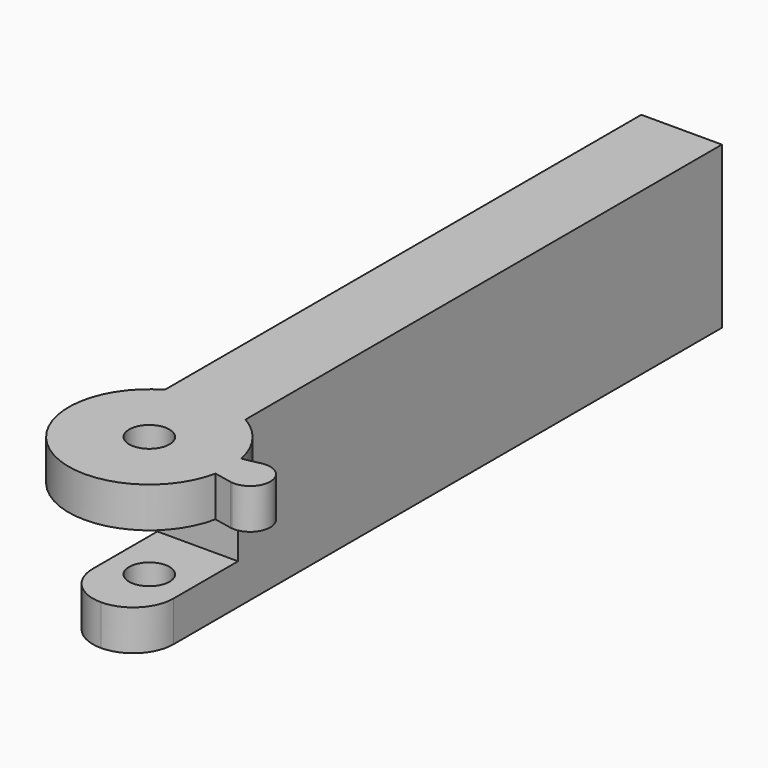
from build123d import *

# Parameters (mm, degrees)
F0_W      = 12.7
F0_H      = 114.3
F1_DEPTH  = 25.4
F2_W      = 19.05
F2_H      = 12.7
F3_DEPTH  = 12.701
F4_R      = 6.34999
F5_R      = 3.175
F6_DEPTH  = 25.401
F8_DEPTH  = 6.35
F10_DEPTH = 6.35


# Not quite as in the source:
# - a fillet or chamfer is up to 0.001 mm smaller than in the source, because OpenCascade refuses the exact size


with BuildPart() as f1:
    # F0 (on Top) → F1 (new body)
    with BuildSketch(Plane.XY):
        with Locations((6.35, 57.15)):
            Rectangle(F0_W, F0_H)
    extrude(amount=F1_DEPTH)

    # F2 (on face) → F3 (cut, through all)
    with BuildSketch(Plane.YZ.offset(12.7)):
        with Locations((9.525, 12.7)):
            Rectangle(F2_W, F2_H)
    extrude(amount=-F3_DEPTH, mode=Mode.SUBTRACT)

    # F4 (radius 6.35 in the source; OpenCascade refuses exactly that, so slightly less here)
    f4_edges = [f1.edges().sort_by_distance(p)[0] for p in [
        (12.7, 0, 22.225),
        (12.7, 0, 3.175),
        (0, 0, 3.175),
        (0, 0, 22.225),
    ]]
    fillet(f4_edges, radius=F4_R)

    # F5 (on face) → F6 (cut, through all)
    with BuildSketch(Plane.XY.offset(25.4)):
        with Locations((6.35, 9.525)):
            Circle(F5_R)
    extrude(amount=-F6_DEPTH, mode=Mode.SUBTRACT)

    # F7 (on face) → F8 (join, through all)
    with BuildSketch(Plane.XY.offset(25.4)):
        with BuildLine():
            Line((0, 6.35), (0, 20.5235226281))
            ThreePointArc((0, 20.5235226281), (6.35, -3.175), (12.7, 20.5235226281))
            Line((12.7, 20.5235226281), (12.7, 6.35))
            ThreePointArc((12.7, 6.35), (6.35, 0), (0, 6.35))
        make_face()
    extrude(amount=-F8_DEPTH)

    # F9 (on face) → F10 (join, through all)
    with BuildSketch(Plane.XY.offset(25.4)):
        with BuildLine():
            ThreePointArc((21.59, 12.6358519733), (21.7481397779, 12.663985398), (21.9075, 12.6840851128))
            ThreePointArc((21.9075, 12.6840851128), (21.9058819686, 12.6920429708), (21.9042598667, 12.7))
            Line((21.9042598667, 12.7), (21.59, 12.6358519733))
        make_face()
        with BuildLine():
            ThreePointArc((21.9075, 6.3659148872), (25.4, 9.525), (21.9075, 12.6840851128))
            ThreePointArc((21.9075, 12.6840851128), (21.7481397779, 12.663985398), (21.59, 12.6358519733))
            Line((21.59, 12.6358519733), (18.7934078933, 12.065))
            ThreePointArc((18.7934078933, 12.065), (19.05, 9.525), (18.7934078933, 6.985))
            Line((18.7934078933, 6.985), (21.59, 6.4141480267))
            ThreePointArc((21.59, 6.4141480267), (21.7481397779, 6.386014602), (21.9075, 6.3659148872))
        make_face()
        with BuildLine():
            ThreePointArc((21.9042598667, 6.35), (21.9058819686, 6.3579570292), (21.9075, 6.3659148872))
            ThreePointArc((21.9075, 6.3659148872), (21.7481397779, 6.386014602), (21.59, 6.4141480267))
            Line((21.59, 6.4141480267), (21.9042598667, 6.35))
        make_face()
    extrude(amount=-F10_DEPTH)


solid = f1.part
